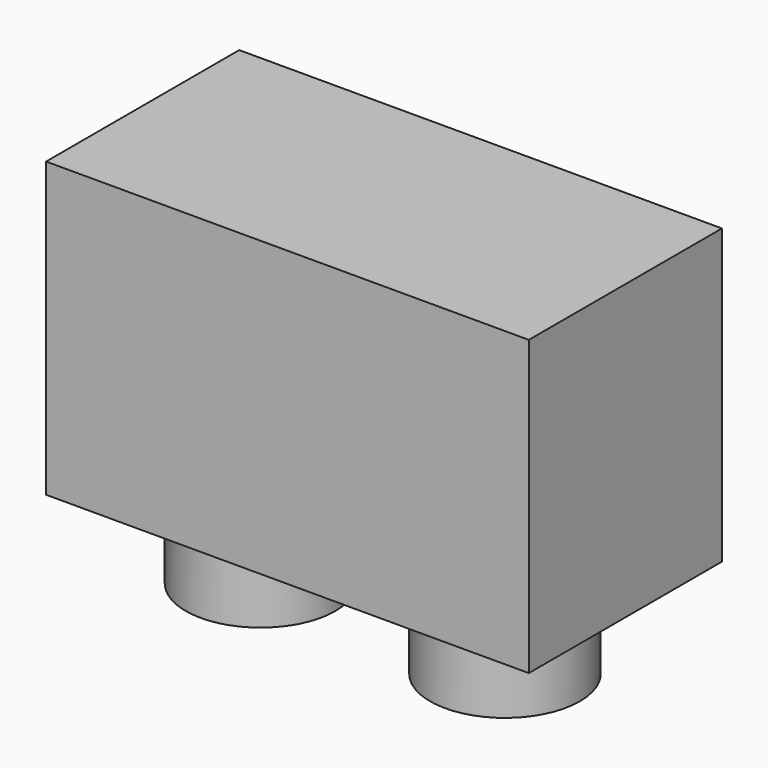
from build123d import *

# Parameters (mm, degrees)
F0_W     = 15.7988
F0_H     = 7.8994
F0_R     = 2.44983
F1_DEPTH = 9.6012
F2_DEPTH = 2.8702


# Not quite as in the source:
# - a feature names something its author has since deleted; it is built from what else it names


with BuildPart() as f1:
    # F0 (on Top) → F1 (new body)
    with BuildSketch(Plane.XY):
        with Locations((-7.8994, -3.9497)):
            Rectangle(F0_W, F0_H)
        with Locations((-11.89863, -3.99923)):
            Circle(F0_R, mode=Mode.SUBTRACT)
        with Locations((-3.90017, -3.99923)):
            Circle(F0_R, mode=Mode.SUBTRACT)
        with Locations((-11.89863, -3.99923)):
            Circle(F0_R)
        with Locations((-3.90017, -3.99923)):
            Circle(F0_R)
    extrude(amount=F1_DEPTH)

    # F0 (on Top) → F2 (join)
    with BuildSketch(Plane.XY):
        with Locations((-3.90017, -3.99923)):
            Circle(F0_R)
        with Locations((-11.89863, -3.99923)):
            Circle(F0_R)
    extrude(amount=-F2_DEPTH)


solid = f1.part
